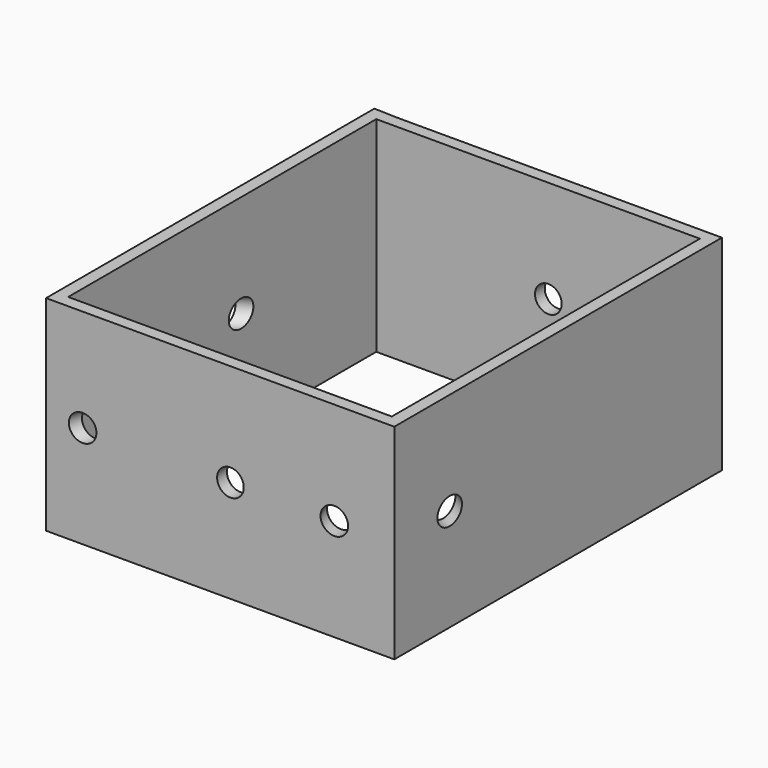
from build123d import *

# Parameters (mm, degrees)
F2_DEPTH  = 25
F3_DEPTH  = 25
F10_R     = 3.25
F11_DEPTH = 50
F12_R     = 3.25
F13_DEPTH = 50
F14_R     = 3.25
F15_DEPTH = 120
F22_R     = 3.25
F23_DEPTH = 100
F24_R     = 3.25
F25_DEPTH = 100


with BuildPart() as f2:
    # F1 (on Top) → F2 (new body)
    with BuildSketch(Plane.XY):
        Polygon((-45, -60), (-40, -60), (40, -60), (40, 39.9669196701), (-36.0033019851, 39.9669196701), (-39.0033019851, 39.9669196701), (-42.0016509926, 40.0664346415), (-45, 40.1659496129), align=None)
        Polygon((37, -57), (-37, -57), (-42.0016509926, -57), (-42.0016509926, 37), (-37, 37), (37, 37), align=None, mode=Mode.SUBTRACT)
    extrude(amount=F2_DEPTH)

    # F1 (on Top) → F3 (join)
    with BuildSketch(Plane.XY):
        Polygon((-45, -60), (-40, -60), (40, -60), (40, 39.9669196701), (-36.0033019851, 39.9669196701), (-39.0033019851, 39.9669196701), (-42.0016509926, 40.0664346415), (-45, 40.1659496129), align=None)
        Polygon((37, -57), (-37, -57), (-42.0016509926, -57), (-42.0016509926, 37), (-37, 37), (37, 37), align=None, mode=Mode.SUBTRACT)
    extrude(amount=-F3_DEPTH)

    # F10 (on face) → F11 (cut)
    with BuildSketch(Plane(origin=(8.6602540378, -32.3205080757, 0), x_dir=(-0.9659258263, -0.2588190451, 0), z_dir=(-0.2588190451, 0.9659258263, 0))):
        with Locations((-8.9657547217, 0)):
            Circle(F10_R)
    extrude(amount=-F11_DEPTH, mode=Mode.SUBTRACT)

    # F12 (on face) → F13 (cut)
    with BuildSketch(Plane(origin=(25.9807621135, -15, 0), x_dir=(0.5, 0.8660254038, 0), z_dir=(0.8660254038, -0.5, 0))):
        with Locations((-17.3205080757, 0)):
            Circle(F12_R)
    extrude(amount=F13_DEPTH, mode=Mode.SUBTRACT)

    # F14 (on face) → F15 (cut)
    with BuildSketch(Plane.XZ.offset(60)):
        Circle(F14_R)
    extrude(amount=-F15_DEPTH, mode=Mode.SUBTRACT)

    # F22 (on face) → F23 (cut)
    with BuildSketch(Plane(origin=(1.3397459622, 5, 0), x_dir=(0.9659258263, -0.2588190451, 0), z_dir=(-0.2588190451, -0.9659258263, 0))):
        with Locations((-19.3185165258, 0)):
            Circle(F22_R)
    extrude(amount=F23_DEPTH, mode=Mode.SUBTRACT)

    # F24 (on face) → F25 (cut)
    with BuildSketch(Plane(origin=(-8.6602540378, -5, 0), x_dir=(-0.5, 0.8660254038, 0), z_dir=(0.8660254038, 0.5, 0))):
        with Locations((17.3205080757, 0)):
            Circle(F24_R)
    extrude(amount=-F25_DEPTH, mode=Mode.SUBTRACT)


solid = f2.part
